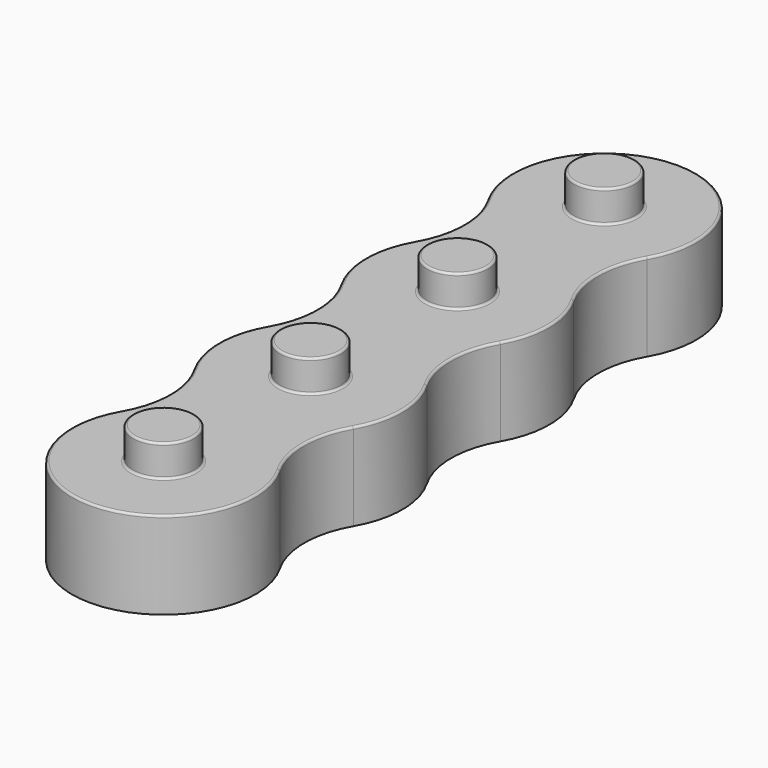
from build123d import *

# Parameters (mm, degrees)
F4_R     = 7.9
F5_DEPTH = 20
F6_DEPTH = 10
F7_R     = 7
F8_DEPTH = 7.3
F9_R     = 0.5


# Not quite as in the source:
# - a feature names something its author has since deleted; it is built from what else it names


with BuildPart() as f5:
    # F4 (on Top) → F5 (new body)
    with BuildSketch(Plane.XY):
        with BuildLine():
            ThreePointArc((18.1865334795, 10.5), (15.3730669589, 21), (18.1865334795, 31.5))
            ThreePointArc((18.1865334795, 31.5), (21, 42), (18.1865334795, 52.5))
            ThreePointArc((18.1865334795, 52.5), (15.3730669589, 63), (18.1865334795, 73.5))
            ThreePointArc((18.1865334795, 73.5), (21, 84), (18.1865334795, 94.5))
            ThreePointArc((18.1865334795, 94.5), (15.3730669589, 105), (18.1865334795, 115.5))
            ThreePointArc((18.1865334795, 115.5), (0, 147), (-18.1865334795, 115.5))
            ThreePointArc((-18.1865334795, 115.5), (-15.3730669589, 105), (-18.1865334795, 94.5))
            ThreePointArc((-18.1865334795, 94.5), (-21, 84), (-18.1865334795, 73.5))
            ThreePointArc((-18.1865334795, 73.5), (-15.3730669589, 63), (-18.1865334795, 52.5))
            ThreePointArc((-18.1865334795, 52.5), (-21, 42), (-18.1865334795, 31.5))
            ThreePointArc((-18.1865334795, 31.5), (-15.3730669589, 21), (-18.1865334795, 10.5))
            ThreePointArc((-18.1865334795, 10.5), (0, -21), (18.1865334795, 10.5))
        make_face()
        Circle(F4_R, mode=Mode.SUBTRACT)
        with Locations((0, 42)):
            Circle(F4_R, mode=Mode.SUBTRACT)
        with Locations((0, 84)):
            Circle(F4_R, mode=Mode.SUBTRACT)
        with Locations((0, 126)):
            Circle(F4_R, mode=Mode.SUBTRACT)
        with Locations((0, 42)):
            Circle(F4_R)
        Circle(F4_R)
        with Locations((0, 126)):
            Circle(F4_R)
        with Locations((0, 84)):
            Circle(F4_R)
    extrude(amount=F5_DEPTH)

    # F4 (on Top) → F6 (cut)
    with BuildSketch(Plane.XY):
        with Locations((0, 42)):
            Circle(F4_R)
        Circle(F4_R)
        with Locations((0, 84)):
            Circle(F4_R)
        with Locations((0, 126)):
            Circle(F4_R)
    extrude(amount=F6_DEPTH, mode=Mode.SUBTRACT)

    # F7 (on face) → F8 (join)
    with BuildSketch(Plane.XY.offset(20)):
        Circle(F7_R)
        with Locations((0, 42)):
            Circle(F7_R)
        with Locations((0, 84)):
            Circle(F7_R)
        with Locations((0, 126)):
            Circle(F7_R)
    extrude(amount=F8_DEPTH)

    # F9
    f9_edges = [f5.edges().sort_by_distance(p)[0] for p in [
        (-7, 0, 27.3),
        (-7.9, 42, 0),
        (-7.9, 42, 10),
        (-7.9, 0, 0),
        (-7.9, 0, 10),
        (-7, 42, 27.3),
        (-7, 42, 20),
        (21, 42, 20),
        (-7, 84, 27.3),
        (-7, 84, 20),
        (-7, 126, 27.3),
        (-7, 126, 20),
        (-7.9, 84, 10),
        (-7.9, 84, 0),
        (-7.9, 126, 10),
        (-7.9, 126, 0),
        (-7, 0, 20),
    ]]
    fillet(f9_edges, radius=F9_R)


solid = f5.part
